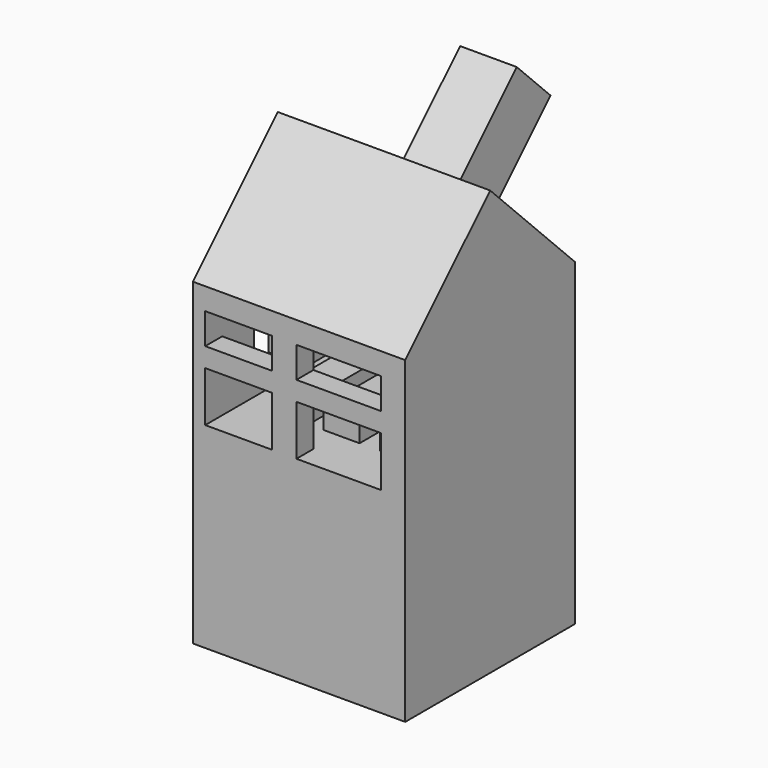
from build123d import *

# Parameters (mm, degrees)
F0_W      = 254
F0_H      = 254
F1_DEPTH  = 508
F2_SIZE   = 127
F3_SIZE   = 126.99999
F4_W      = 110.2521903813
F4_H      = 222.1985608339
F5_DEPTH  = 12.7
F6_R      = 15.2445630658
F7_DEPTH  = 25.4
F8_W      = 60.8862751365
F8_H      = 17.78
F9_DEPTH  = 12.7
F10_W     = 44.4203019142
F10_H     = 51.6851246357
F10_W_2   = 47.3152212799
F10_H_2   = 46.0566580296
F10_W_3   = 41.5758583695
F10_H_3   = 51.8873212337
F10_W_4   = 40.2868166566
F10_H_4   = 50.077855587
F11_DEPTH = 25.4
F12_W     = 67.7322521806
F12_H     = 71.3757276535
F13_DEPTH = 127
F14_W     = 210.3085294366
F14_H     = 119.9935823679
F15_DEPTH = 228.6
F16_W     = 37.6376099885
F16_H     = 126.9762441516
F16_W_2   = 43.185967952
F16_H_2   = 134.4709768891
F16_W_3   = 35.2269485593
F16_H_3   = 143.0262625217
F17_DEPTH = 25.4
F18_R     = 26.1262901257
F18_R_2   = 20.0737439282
F18_R_3   = 29.9342227193
F19_DEPTH = 12.7
F20_W     = 29.2137209326
F20_H     = 63.1077764034
F20_H_2   = 23.1252685189
F20_W_2   = 94.6274452358
F20_W_3   = 130.1588338315
F20_H_3   = 76.8547430634
F21_DEPTH = 25.4


# Not quite as in the source:
# - a fillet or chamfer is up to 0.001 mm smaller than in the source, because OpenCascade refuses the exact size


with BuildPart() as f1:
    # F0 (on Top) → F1 (new body)
    with BuildSketch(Plane.XY):
        with Locations((3.1588338315, -4.6172558538)):
            Rectangle(F0_W, F0_H)
    extrude(amount=F1_DEPTH)

    # F2
    f2_edges = [f1.edges().sort_by_distance(p)[0] for p in [
        (3.158834, -131.617256, 508),
    ]]
    chamfer(f2_edges, length=F2_SIZE)

    # F3 (size 127 in the source; OpenCascade refuses exactly that, so slightly less here)
    f3_edges = [f1.edges().sort_by_distance(p)[0] for p in [
        (3.158834, 122.382744, 508),
    ]]
    chamfer(f3_edges, length=F3_SIZE)

    # F4 (on face) → F5 (join)
    with BuildSketch(Plane(origin=(-123.8411661685, 0, 0), x_dir=(0, -1, 0), z_dir=(-1, 0, 0))):
        with Locations((3.7376638502, 111.099280417)):
            Rectangle(F4_W, F4_H)
    extrude(amount=F5_DEPTH)

    # F6 (on face) → F7 (join)
    with BuildSketch(Plane(origin=(-136.5411661685, 0, 0), x_dir=(0, -1, 0), z_dir=(-1, 0, 0))):
        with Locations((41.2117242813, 101.0684147477)):
            Circle(F6_R)
    extrude(amount=F7_DEPTH)

    # F8 (on face) → F9 (join)
    with BuildSketch(Plane(origin=(-161.9411661685, 0, 0), x_dir=(0, -1, 0), z_dir=(-1, 0, 0))):
        with Locations((22.795823104, 100.5913294025)):
            Rectangle(F8_W, F8_H)
    extrude(amount=F9_DEPTH)

    # F10 (on face) → F11 (cut)
    with BuildSketch(Plane(origin=(-123.8411661685, 0, 0), x_dir=(0, -1, 0), z_dir=(-1, 0, 0))):
        with Locations((-22.2101509571, 357.1109622717)):
            Rectangle(F10_W, F10_H)
        with Locations((-23.6576106399, 284.112855792)):
            Rectangle(F10_W_2, F10_H_2)
        with Locations((38.0553556606, 355.0563393831)):
            Rectangle(F10_W_3, F10_H_3)
        with Locations((38.7203507125, 285.8152091503)):
            Rectangle(F10_W_4, F10_H_4)
    extrude(amount=-F11_DEPTH, mode=Mode.SUBTRACT)

    # F12 (on face) → F13 (join)
    with BuildSketch(Plane(origin=(0, 251.6913720731, 251.6913720731), x_dir=(-1, 0, 0), z_dir=(0, 0.7071067812, 0.7071067812))):
        with Locations((-33.8661260903, 287.2642278671)):
            Rectangle(F12_W, F12_H)
    extrude(amount=F13_DEPTH)

    # F14 (on face) → F15 (cut)
    with BuildSketch(Plane.XZ.offset(131.6172558538)):
        with Locations((-3.9455778897, 294.7669550776)):
            Rectangle(F14_W, F14_H)
    extrude(amount=-F15_DEPTH, mode=Mode.SUBTRACT)

    # F16 (on face) → F17 (join)
    with BuildSketch(Plane.XY.offset(234.7701638937)):
        with Locations((-53.3800702542, -6.8131200969)):
            Rectangle(F16_W, F16_H)
        with Locations((4.870776087, -3.0657537282)):
            Rectangle(F16_W_2, F16_H_2)
        with Locations((68.4281103313, 1.2118890882)):
            Rectangle(F16_W_3, F16_H_3)
    extrude(amount=F17_DEPTH)

    # F18 (on face) → F19 (join)
    with BuildSketch(Plane.XY.offset(260.1701638937)):
        with Locations((-53.3800702542, 75.6483599544)):
            Circle(F18_R)
        with Locations((0, 86.5157917142)):
            Circle(F18_R_2)
        with Locations((55.7353012264, 86.5157917142)):
            Circle(F18_R_3)
    extrude(amount=F19_DEPTH)

    # F20 (on face) → F21 (join)
    with BuildSketch(Plane.XZ.offset(131.6172558538)):
        with Locations((-14.6068604663, 349.4461117983)):
            Rectangle(F20_W, F20_H)
        with Locations((-14.6068604663, 306.3295893371)):
            Rectangle(F20_W, F20_H_2)
        with Locations((-76.5274435505, 306.3295893371)):
            Rectangle(F20_W_2, F20_H_2)
        with Locations((65.0794169158, 306.3295893371)):
            Rectangle(F20_W_3, F20_H_2)
        with Locations((-14.6068604663, 256.3395835459)):
            Rectangle(F20_W, F20_H_3)
    extrude(amount=-F21_DEPTH)


solid = f1.part
